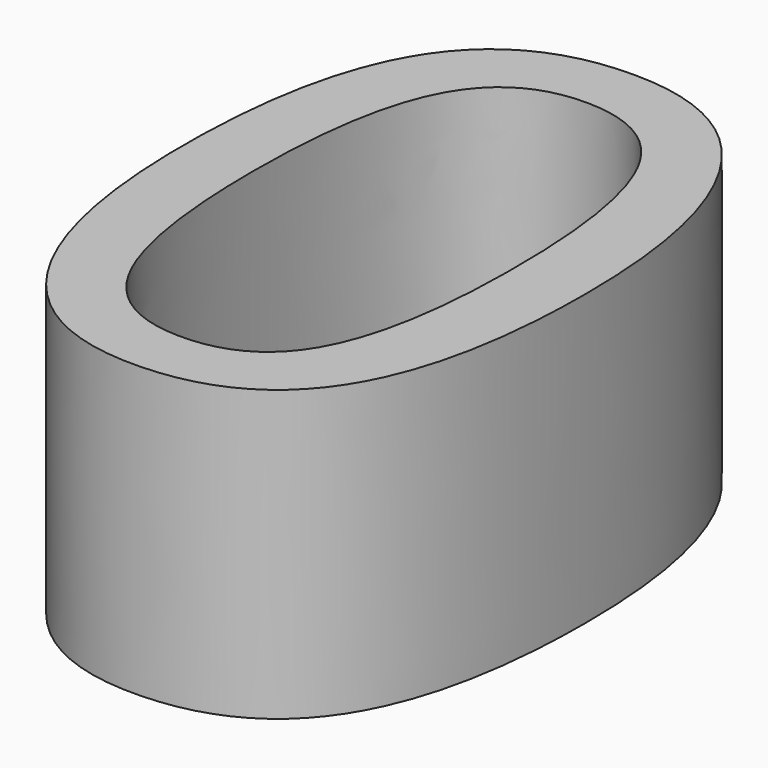
from build123d import *

# Parameters (mm, degrees)
F0_TEXT_SIZE = 8.8194444444
F1_DEPTH     = 2.9972


# Not quite as in the source:
# - Text() gives the source's letters only with a copy of the font that has no kerning and outlines rounded to 1/6400 em; it was checked with that copy


with BuildPart() as f1:
    # F0 (on Top) → F1 (new body)
    with BuildSketch(Plane.XY):
        with Locations((-3.3678137778, -3.8691295556)):
            Text('0', F0_TEXT_SIZE, font='Open Sans', text_align=(TextAlign.LEFT, TextAlign.BOTTOM))
    extrude(amount=F1_DEPTH)


solid = f1.part
